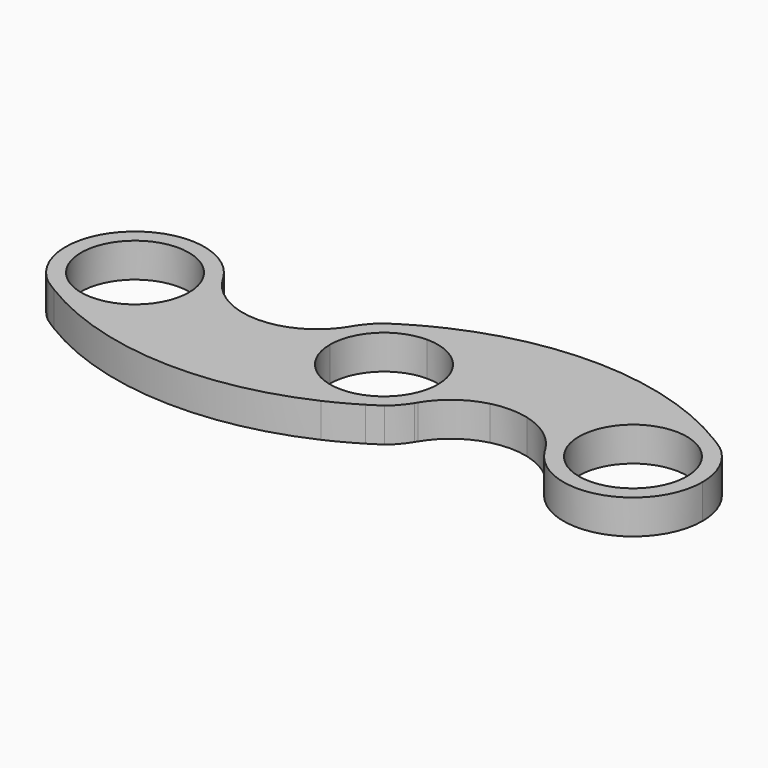
from build123d import *

# Parameters (mm, degrees)
F0_R     = 11
F1_DEPTH = 7


with BuildPart() as f1:
    # F0 (on Top) → F1 (new body)
    with BuildSketch(Plane.XY):
        with BuildLine():
            Line((14.175, 0), (11, 0))
            ThreePointArc((11, 0), (7.7781745931, -7.7781745931), (0, -11))
            Line((0, -11), (0, -14.175))
            ThreePointArc((0, -14.175), (3.2814696071, -13.7899449679), (6.3846610647, -12.655699431))
            ThreePointArc((6.3846610647, -12.655699431), (7.6740188796, -11.8429761162), (8.9426071008, -10.9982))
            ThreePointArc((8.9426071008, -10.9982), (10.6919977036, -9.3065466262), (12.1262614453, -7.3406))
            ThreePointArc((12.1262614453, -7.3406), (12.2596266851, -7.1057126256), (12.3971479741, -6.8732341084))
            ThreePointArc((12.3971479741, -6.8732341084), (13.7233413849, -3.5497219939), (14.175, 0))
        make_face()
        with BuildLine():
            ThreePointArc((0, 11), (7.7781745931, 7.7781745931), (11, 0))
            Line((11, 0), (14.175, 0))
            ThreePointArc((14.175, 0), (10.0232386233, 10.0232386233), (0, 14.175))
            Line((0, 14.175), (0, 11))
        make_face()
        with BuildLine():
            ThreePointArc((-11, 0), (-7.7781745931, 7.7781745931), (0, 11))
            Line((0, 11), (0, 14.175))
            ThreePointArc((0, 14.175), (-3.2888623779, 13.7881836824), (-6.3982276645, 12.6488461036))
            ThreePointArc((-6.3982276645, 12.6488461036), (-7.6795852422, 11.8402648338), (-8.9403928885, 11))
            ThreePointArc((-8.9403928885, 11), (-10.6938487189, 9.304419626), (-12.1306573285, 7.3333333333))
            ThreePointArc((-12.1306573285, 7.3333333333), (-12.2610462299, 7.103700791), (-12.3954086387, 6.8763703856))
            ThreePointArc((-12.3954086387, 6.8763703856), (-13.7228922326, 3.5514579785), (-14.175, 0))
            Line((-14.175, 0), (-11, 0))
        make_face()
        with BuildLine():
            Line((0, -14.175), (0, -11))
            ThreePointArc((0, -11), (-7.7781745931, -7.7781745931), (-11, 0))
            Line((-11, 0), (-14.175, 0))
            ThreePointArc((-14.175, 0), (-10.0232386233, -10.0232386233), (0, -14.175))
        make_face()
        with BuildLine():
            ThreePointArc((0, 14.175), (10.0232386233, 10.0232386233), (14.175, 0))
            Line((14.175, 0), (21.6662, 0))
            ThreePointArc((21.6662, 0), (25.4, 0.4661082384), (29.1338, 0))
            Line((29.1338, 0), (36.625, 0))
            ThreePointArc((36.625, 0), (43.3747333645, 12.0746031153), (57.1958698966, 12.650038469))
            ThreePointArc((57.1958698966, 12.650038469), (29.0258725789, 21.5203456529), (0, 16.0678398574))
            Line((0, 16.0678398574), (0, 14.175))
        make_face()
        with BuildLine():
            Line((21.6662, 0), (14.175, 0))
            ThreePointArc((14.175, 0), (13.7233413849, -3.5497219939), (12.3971479741, -6.8732341084))
            ThreePointArc((12.3971479741, -6.8732341084), (16.353496972, -2.5220464261), (21.6662, 0))
        make_face()
        with BuildLine():
            ThreePointArc((-6.3982276645, 12.6488461036), (-3.2888623779, 13.7881836824), (0, 14.175))
            Line((0, 14.175), (0, 16.0678398574))
            ThreePointArc((0, 16.0678398574), (-3.2501607804, 14.453871086), (-6.3982276645, 12.6488461036))
        make_face()
        with BuildLine():
            Line((0, -16.0641572656), (0, -14.175))
            ThreePointArc((0, -14.175), (-10.0232386233, -10.0232386233), (-14.175, 0))
            Line((-14.175, 0), (-21.6559333333, 0))
            ThreePointArc((-21.6559333333, 0), (-25.4, -0.4688166689), (-29.1440666667, 0))
            Line((-29.1440666667, 0), (-36.625, 0))
            ThreePointArc((-36.625, 0), (-43.3693858125, -12.0713130104), (-57.1846610647, -12.655699431))
            ThreePointArc((-57.1846610647, -12.655699431), (-29.0187526069, -21.5141320936), (0, -16.0641572656))
        make_face()
        with BuildLine():
            ThreePointArc((6.3846610647, -12.655699431), (3.2814696071, -13.7899449679), (0, -14.175))
            Line((0, -14.175), (0, -16.0641572656))
            ThreePointArc((0, -16.0641572656), (3.2430752796, -14.4549824836), (6.3846610647, -12.655699431))
        make_face()
        with BuildLine():
            Line((-21.6559333333, 0), (-14.175, 0))
            ThreePointArc((-14.175, 0), (-13.7228922326, 3.5514579785), (-12.3954086387, 6.8763703856))
            ThreePointArc((-12.3954086387, 6.8763703856), (-16.3473482418, 2.5246764417), (-21.6559333333, 0))
        make_face()
        with BuildLine():
            Line((36.625, 0), (29.1338, 0))
            ThreePointArc((29.1338, 0), (34.446503028, -2.5220464261), (38.4028520259, -6.8732341084))
            ThreePointArc((38.4028520259, -6.8732341084), (37.0766586151, -3.5497219939), (36.625, 0))
        make_face()
        with BuildLine():
            ThreePointArc((59.7426071008, 10.9982), (58.47955068, 11.8400181351), (57.1958698966, 12.650038469))
            ThreePointArc((57.1958698966, 12.650038469), (43.3747333645, 12.0746031153), (36.625, 0))
            ThreePointArc((36.625, 0), (37.0766586151, -3.5497219939), (38.4028520259, -6.8732341084))
            ThreePointArc((38.4028520259, -6.8732341084), (38.5403733149, -7.1057126256), (38.6737385547, -7.3406))
            ThreePointArc((38.6737385547, -7.3406), (54.6105687904, -13.6532117281), (64.975, 0))
            ThreePointArc((64.975, 0), (63.6002359481, 6.0897113784), (59.7426071008, 10.9982))
        make_face()
        with BuildLine():
            ThreePointArc((61.8, 0), (50.8, -11), (39.8, 0))
            ThreePointArc((39.8, 0), (50.8, 11), (61.8, 0))
        make_face(mode=Mode.SUBTRACT)
        with BuildLine():
            ThreePointArc((-59.7426071008, -10.9982), (-58.4740188796, -11.8429761162), (-57.1846610647, -12.655699431))
            ThreePointArc((-57.1846610647, -12.655699431), (-43.3693858125, -12.0713130104), (-36.625, 0))
            ThreePointArc((-36.625, 0), (-37.0771077674, 3.5514579785), (-38.4045913613, 6.8763703856))
            ThreePointArc((-38.4045913613, 6.8763703856), (-38.5389537701, 7.103700791), (-38.6693426715, 7.3333333333))
            ThreePointArc((-38.6693426715, 7.3333333333), (-60.1033431975, 10.6947851941), (-59.7426071008, -10.9982))
        make_face()
        with Locations((-50.8, 0)):
            Circle(F0_R, mode=Mode.SUBTRACT)
        with BuildLine():
            Line((-36.625, 0), (-29.1440666667, 0))
            ThreePointArc((-29.1440666667, 0), (-34.4526517582, 2.5246764417), (-38.4045913613, 6.8763703856))
            ThreePointArc((-38.4045913613, 6.8763703856), (-37.0771077674, 3.5514579785), (-36.625, 0))
        make_face()
    extrude(amount=F1_DEPTH)


solid = f1.part
